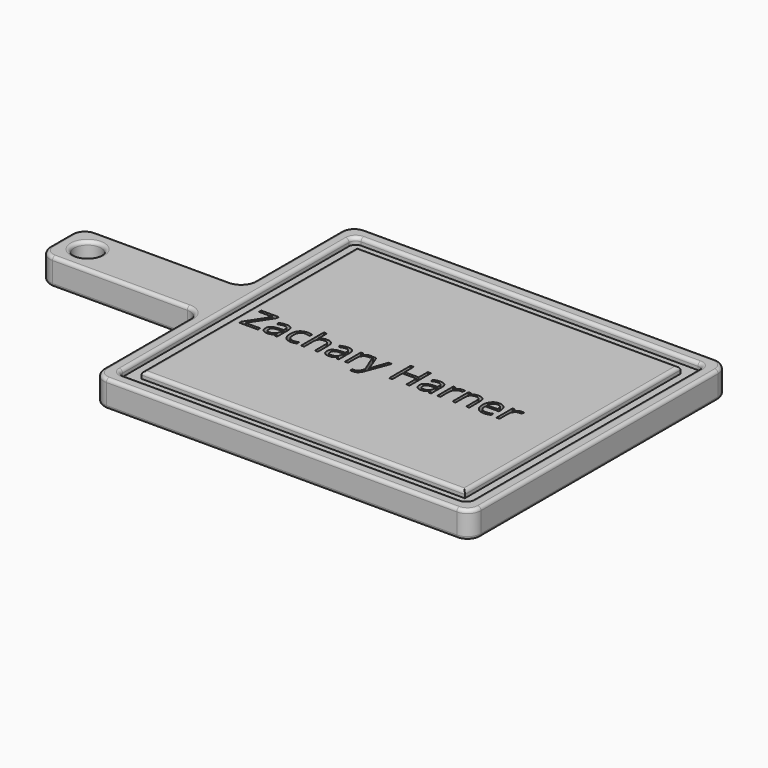
from build123d import *

# Parameters (mm, degrees)
F0_W         = 152.4
F0_H         = 50.8
F1_DEPTH     = 25.4
F2_R         = 12.7
F3_DEPTH     = 25.4
F5_DEPTH     = 6.35
F6_R         = 6.35
F7_R         = 12.7
F8_R         = 3.175
F9_TEXT_SIZE = 35.2777777778
F10_DEPTH    = 5.08


# Not quite as in the source:
# - Text() gives the source's letters only with a copy of the font that has no kerning and outlines rounded to 1/6400 em; it was checked with that copy


with BuildPart() as f1:
    # F0 (on Top) → F1 (new body)
    with BuildSketch(Plane.XY):
        Polygon((0, 127), (0, 0), (355.6, 0), (355.6, 304.8), (0, 304.8), (0, 177.8), align=None)
        with Locations((-76.2, 152.4)):
            Rectangle(F0_W, F0_H)
    extrude(amount=F1_DEPTH)

    # F2 (on face) → F3 (cut)
    with BuildSketch(Plane.XY.offset(25.4)):
        with Locations((-127, 152.4)):
            Circle(F2_R)
    extrude(amount=-F3_DEPTH, mode=Mode.SUBTRACT)

    # F4 (on face) → F5 (cut)
    with BuildSketch(Plane.XY.offset(25.4)):
        Polygon((12.6999876976, 127), (12.6999876976, 12.6999876976), (342.9000123024, 12.6999876976), (342.9000123024, 292.1000123024), (12.6999876976, 292.1000123024), (12.6999876976, 177.8), align=None)
        Polygon((25.3999791622, 127), (25.3999791622, 177.8), (25.3999791622, 279.4000208378), (330.2000208378, 279.4000208378), (330.2000208378, 25.3999791622), (25.3999791622, 25.3999791622), align=None, mode=Mode.SUBTRACT)
    extrude(amount=-F5_DEPTH, mode=Mode.SUBTRACT)

    # F6
    f6_edges = [f1.edges().sort_by_distance(p)[0] for p in [
        (12.699988, 292.100012, 22.225),
        (342.900012, 292.100012, 22.225),
        (342.900012, 12.699988, 22.225),
        (12.699988, 12.699988, 22.225),
    ]]
    fillet(f6_edges, radius=F6_R)

    # F7
    f7_edges = [f1.edges().sort_by_distance(p)[0] for p in [
        (-152.4, 127, 12.7),
        (0, 127, 12.7),
        (-152.4, 177.8, 12.7),
        (0, 177.8, 12.7),
        (0, 304.8, 12.7),
        (355.6, 304.8, 12.7),
        (355.6, 0, 12.7),
        (0, 0, 12.7),
    ]]
    fillet(f7_edges, radius=F7_R)

    # F8
    f8_edges = [f1.edges().sort_by_distance(p)[0] for p in [
        (177.8, 279.400021, 25.4),
        (330.200021, 152.4, 25.4),
        (177.8, 25.399979, 25.4),
        (25.399979, 152.4, 25.4),
        (0, 63.5, 25.4),
        (-3.719744, 123.280256, 25.4),
        (3.719744, 3.719744, 25.4),
        (-76.2, 127, 25.4),
        (177.8, 0, 25.4),
        (-148.680256, 130.719744, 25.4),
        (351.880256, 3.719744, 25.4),
        (-152.4, 152.4, 25.4),
        (355.6, 152.4, 25.4),
        (-148.680256, 174.080256, 25.4),
        (351.880256, 301.080256, 25.4),
        (-76.2, 177.8, 25.4),
        (177.8, 304.8, 25.4),
        (-3.719744, 181.519744, 25.4),
        (3.719744, 301.080256, 25.4),
        (0, 241.3, 25.4),
        (177.8, 12.699988, 25.4),
        (14.55986, 14.55986, 25.4),
        (341.04014, 14.55986, 25.4),
        (12.699988, 152.4, 25.4),
        (342.900012, 152.4, 25.4),
        (14.55986, 290.24014, 25.4),
        (341.04014, 290.24014, 25.4),
        (177.8, 292.100012, 25.4),
        (-139.7, 152.4, 25.4),
        (0, 63.5, 0),
        (-3.719744, 123.280256, 0),
        (3.719744, 3.719744, 0),
        (-76.2, 127, 0),
        (177.8, 0, 0),
        (-148.680256, 130.719744, 0),
        (351.880256, 3.719744, 0),
        (-152.4, 152.4, 0),
        (355.6, 152.4, 0),
        (-148.680256, 174.080256, 0),
        (351.880256, 301.080256, 0),
        (-76.2, 177.8, 0),
        (177.8, 304.8, 0),
        (-3.719744, 181.519744, 0),
        (3.719744, 301.080256, 0),
        (0, 241.3, 0),
        (-139.7, 152.4, 0),
    ]]
    fillet(f8_edges, radius=F8_R)

    # F9 (on face) → F10 (cut)
    with BuildSketch(Plane.XY.offset(25.4)):
        with Locations((32.044455442, 130.7452584407)):
            Text('Zachary Harner', F9_TEXT_SIZE, font='Open Sans', text_align=(TextAlign.LEFT, TextAlign.BOTTOM))
    extrude(amount=-F10_DEPTH, mode=Mode.SUBTRACT)


solid = f1.part
